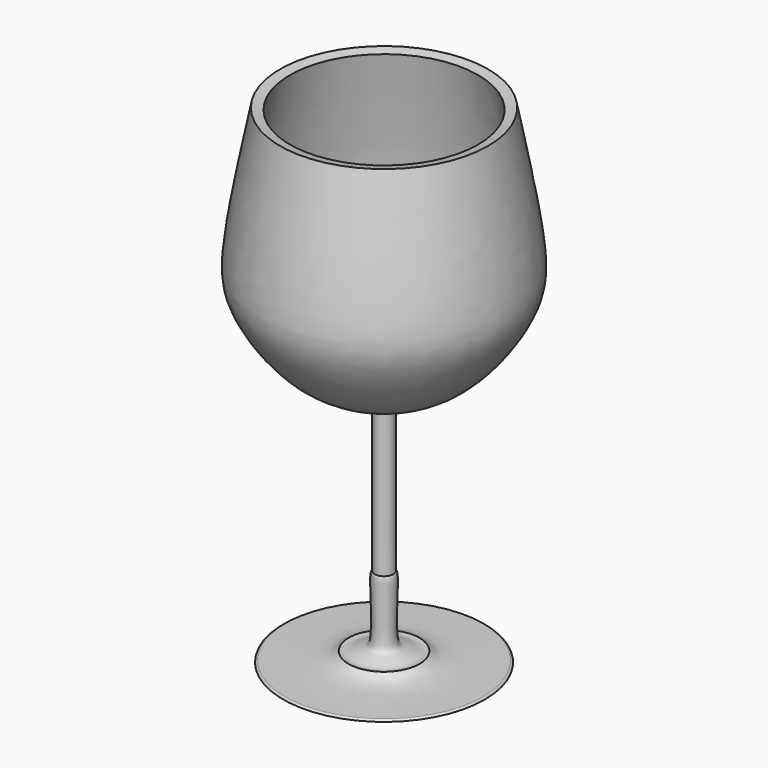
from build123d import *


# Not quite as in the source:
# - a fillet or chamfer that OpenCascade refuses, or shapes differently, is made with other operations: its cross-section is extruded or revolved along the edge and cut away or added
# - the dataset's text gives a spline's control points without its knots; the knots are read off the source's solid


with BuildPart() as f1:
    # F0 (on Front) → F1 (revolve)
    with BuildSketch(Plane.XZ):
        with BuildLine():
            Line((0, 60.6835215705), (0, 0))
            Line((0, 0), (25.4, 0))
            Line((25.4, 0), (25.3756456077, 0.4506908008))
            add(Edge.make_bspline(
                [(8.920145147, 2.54), (9.5701787059, 2.0238867744), (11.2745971474, 0.6706137203), (18.7436626828, 0.5054067019), (23.1824497694, 0.4687853418), (25.3756456077, 0.4506908008)],
                knots=[0, 0, 0, 0, 0.2377416161, 0.6233696542, 1, 1, 1, 1], degree=3))
            add(Edge.make_bspline(
                [(2.3554746294, 20.3104917891), (3.450805073, 20.0467872615), (1.263569687, 3.4623897189), (4.8323470292, 3.4918212397), (7.4855892325, 2.1088926231), (8.6602480308, 2.4779700202), (8.920145147, 2.54)],
                knots=[0, 0, 0, 0, 0.4681347427, 0.6617738747, 0.8644309645, 1, 1, 1, 1], degree=3))
            Line((2.3554746294, 20.3104917891), (2.3554746294, 58.4104917891))
            add(Edge.make_bspline(
                [(2.3554746294, 58.4104917891), (7.8455436813, 59.8572076751), (19.1769192471, 62.8431958086), (31.7113717173, 80.2910669105), (32.4645570364, 91.6023780933), (28.6348578454, 110.8645085553), (26.2116324157, 123.0525374413)],
                knots=[0, 0, 0, 0, 0.2364598605, 0.4880476839, 0.6760644089, 1, 1, 1, 1], degree=3))
            Line((26.2116324157, 123.0525374413), (23.7203938435, 122.5572290763))
            add(Edge.make_bspline(
                [(1.7082412452, 60.8666450715), (3.1593514466, 61.249034466), (6.0146524571, 62.002165491), (10.1014675931, 63.3350542415), (13.3110327941, 64.7970762789), (15.761949944, 66.2881158141), (17.5421523146, 67.6005493036), (19.3026215128, 69.147153639), (21.5681543069, 71.4426571884), (23.6518886123, 73.9928770332), (25.4418980822, 76.5894956432), (26.6119088932, 78.5063430334), (27.421473176, 80.0306656667), (27.9575559056, 81.1755198233), (28.4141500288, 82.2560217519), (28.8425959179, 83.4954427212), (29.1726397755, 84.8949684895), (29.3540159051, 86.3139000071), (29.4054034162, 87.8604329646), (29.34708925, 89.32802144), (29.2453624673, 90.6421135155), (29.1100473168, 92.0590660568), (28.882501846, 94.001859929), (28.5242406922, 96.5763017262), (28.0902028857, 99.3633710421), (27.4229321443, 103.3256055084), (26.4464362239, 108.6717758599), (25.1222270624, 115.5064401591), (24.1879299634, 120.205675785), (23.7203938435, 122.5572290763)],
                knots=[0, 0, 0, 0, 0.0625, 0.125, 0.1875, 0.21875, 0.25, 0.28125, 0.3125, 0.375, 0.40625, 0.4375, 0.46875, 0.484375, 0.5, 0.53125, 0.5625, 0.59375, 0.625, 0.65625, 0.671875, 0.6875, 0.71875, 0.75, 0.78125, 0.8125, 0.875, 0.9375, 1, 1, 1, 1], degree=3))
            Line((1.7082412452, 60.8666450715), (0, 60.6835215705))
        make_face()
    revolve(axis=Axis((0, 0, 30.3417607852), (0, 0, -1)))

    # F2: fillet of radius 0.508 on 1 edges, made by hand

    # F2_s1 → F2_t2 (revolve, cut)
    with BuildSketch(Plane.XZ):
        with BuildLine():
            ThreePointArc((25.4014014901, -0.0259353087), (25.2450528093, 0.3139752222), (24.8983560519, 0.4546359394))
            ThreePointArc((24.8983560519, 0.4546359394), (25.137000807, 0.4526606135), (25.3756456077, 0.4506908008))
            Line((25.3756456077, 0.4506908008), (25.4014014901, -0.0259353087))
        make_face()
    revolve(axis=Axis((0, 0, 0.4506908008), (0, 0, -1)), mode=Mode.SUBTRACT)


solid = f1.part
